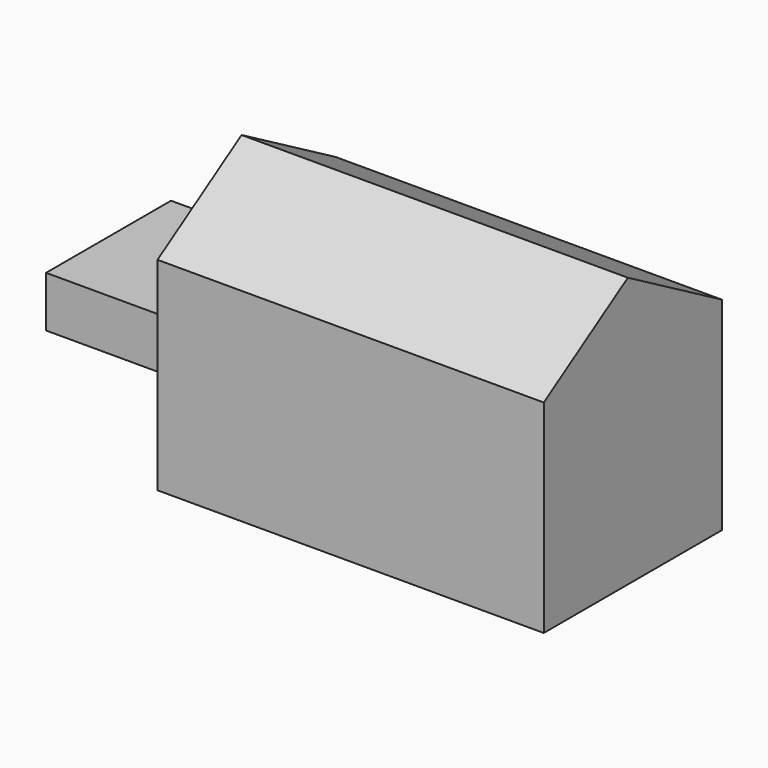
from build123d import *

# Parameters (mm, degrees)
F1_DEPTH = 193.04
F2_W     = 122.8137016296
F2_H     = 78.0344456434
F3_DEPTH = 25.4


# Not quite as in the source:
# - a feature names something its author has since deleted; it is built from what else it names


with BuildPart() as f1:
    # F0 (on Right) → F1 (new body)
    with BuildSketch(Plane.YZ):
        Polygon((-52.5168515742, 56.4679652452), (-52.5168515742, -44.9438914657), (58.7727762759, -44.9438914657), (58.7727762759, 56.4679652452), (0, 90.0208726525), align=None)
    extrude(amount=F1_DEPTH)

    # F2 (on Top) → F3 (join)
    with BuildSketch(Plane.XY):
        with Locations((-2.963334322, -2.6340745389)):
            Rectangle(F2_W, F2_H)
    extrude(amount=F3_DEPTH)


solid = f1.part
